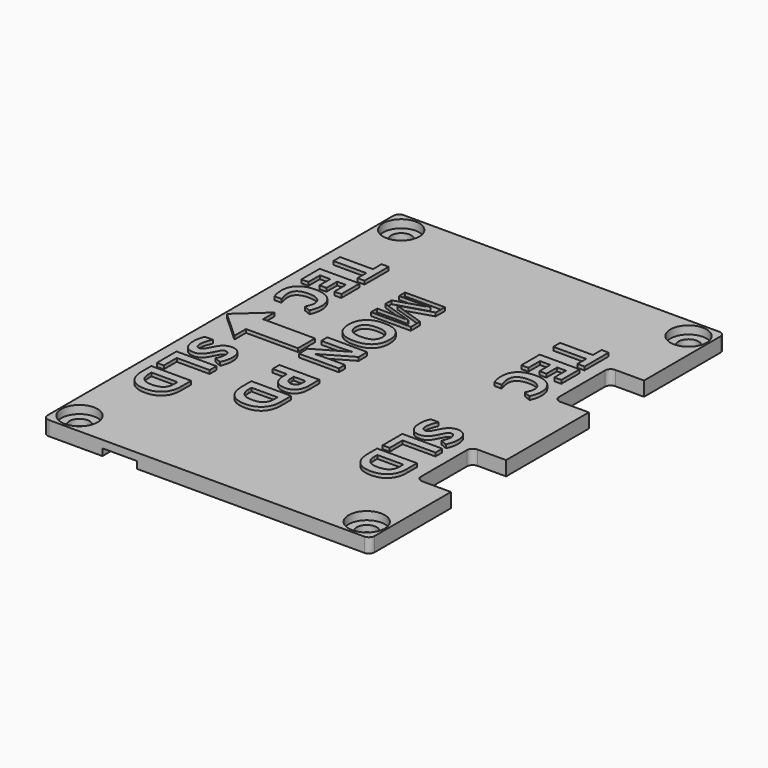
from build123d import *

# Parameters (mm, degrees)
F0_W         = 56.9
F0_H         = 77.2
F0_R         = 1.75
F1_DEPTH     = 2.5
F2_R         = 3.15
F3_DEPTH     = 1.4
F4_W         = 6
F4_H         = 12
F5_DEPTH     = 2.501
F6_TEXT_SIZE = 9.7222222222
F7_DEPTH     = 0.6
F8_R         = 1
F9_W         = 6
F9_H         = 2.5
F10_DEPTH    = 1.2


# Not quite as in the source:
# - Text() gives the source's letters only with a copy of the font that has no kerning and outlines rounded to 1/6400 em; it was checked with that copy


with BuildPart() as f1:
    # F0 (on Top) → F1 (new body)
    with BuildSketch(Plane.XY):
        Rectangle(F0_W, F0_H)
        with Locations((-25, -35)):
            Circle(F0_R, mode=Mode.SUBTRACT)
        with Locations((25, -35)):
            Circle(F0_R, mode=Mode.SUBTRACT)
        with Locations((-25, 35)):
            Circle(F0_R, mode=Mode.SUBTRACT)
        with Locations((25, 35)):
            Circle(F0_R, mode=Mode.SUBTRACT)
    extrude(amount=F1_DEPTH)

    # F2 (on face) → F3 (cut)
    with BuildSketch(Plane.XY.offset(2.5)):
        with Locations((-25, 35)):
            Circle(F2_R)
        with Locations((25, 35)):
            Circle(F2_R)
        with Locations((25, -35)):
            Circle(F2_R)
        with Locations((-25, -35)):
            Circle(F2_R)
    extrude(amount=-F3_DEPTH, mode=Mode.SUBTRACT)

    # F4 (on face) → F5 (cut, through all)
    with BuildSketch(Plane.XY.offset(2.5)):
        with Locations((25.45, 15)):
            Rectangle(F4_W, F4_H)
        with Locations((25.45, -15)):
            Rectangle(F4_W, F4_H)
    extrude(amount=-F5_DEPTH, mode=Mode.SUBTRACT)

    # F6 (on face) → F7 (join)
    with BuildSketch(Plane.XY.offset(2.5)):
        Polygon((-22.5349683315, -1.8524368061), (-15.6800858676, -1.8524368061), (-13.4925916791, -1.8524368061), (-13.4925916791, 0), (-13.4925916791, 1.8524368061), (-15.6800858676, 1.8524368061), (-22.5349683315, 1.8524368061), (-22.5349683315, 4.3779197149), (-27.3454133421, 0), (-22.5349683315, -4.3779197149), align=None)
        with Locations(Location((-25.7820151746, -6.6752677203), (0, 0, -90))):
            Text('SLD', F6_TEXT_SIZE, font='Open Sans', font_style=FontStyle.BOLD, text_align=(TextAlign.LEFT, TextAlign.BOTTOM))
        with Locations(Location((-25.7820151746, 24.7532972845), (0, 0, -90))):
            Text('TEC', F6_TEXT_SIZE, font='Open Sans', font_style=FontStyle.BOLD, text_align=(TextAlign.LEFT, TextAlign.BOTTOM))
        with Locations(Location((-12.3787107544, 20.9212825311), (0, 0, -90))):
            Text('MON PD', F6_TEXT_SIZE, font='Open Sans', font_style=FontStyle.BOLD, text_align=(TextAlign.LEFT, TextAlign.BOTTOM))
        with Locations(Location((13.3408431262, -6.454302423), (0, 0, -90))):
            Text('SLD', F6_TEXT_SIZE, font='Open Sans', font_style=FontStyle.BOLD, text_align=(TextAlign.LEFT, TextAlign.BOTTOM))
        with Locations(Location((13.3408431262, 23.707306286), (0, 0, -90))):
            Text('TEC', F6_TEXT_SIZE, font='Open Sans', font_style=FontStyle.BOLD, text_align=(TextAlign.LEFT, TextAlign.BOTTOM))
    extrude(amount=F7_DEPTH)

    # F8
    f8_edges = [f1.edges().sort_by_distance(p)[0] for p in [
        (22.45, -21, 1.25),
        (22.45, -9, 1.25),
        (22.45, 21, 1.25),
        (22.45, 9, 1.25),
        (28.45, 38.6, 1.25),
        (28.45, -38.6, 1.25),
        (-28.45, -38.6, 1.25),
        (-28.45, 38.6, 1.25),
    ]]
    fillet(f8_edges, radius=F8_R)

    # F9 (on face) → F10 (cut)
    with BuildSketch(Plane(origin=(0, 0, 0), x_dir=(1, 0, 0), z_dir=(0, 0, -1))):
        with Locations((-15.1226357296, 37.35)):
            Rectangle(F9_W, F9_H)
    extrude(amount=-F10_DEPTH, mode=Mode.SUBTRACT)


solid = f1.part
